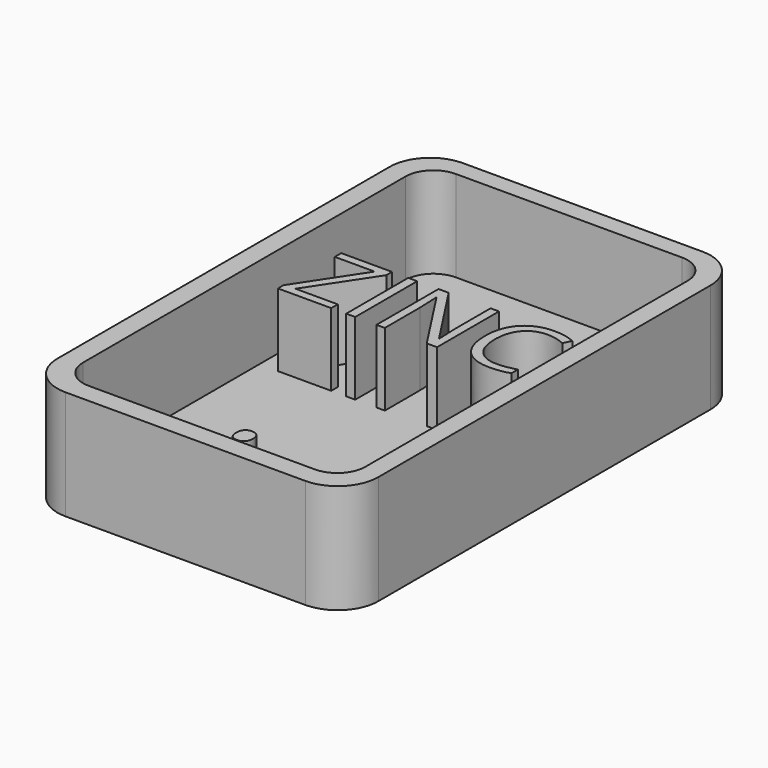
from build123d import *

# Parameters (mm, degrees)
F0_W         = 58.2063253969
F0_H         = 90.0586508214
F1_DEPTH     = 19.812
F2_W         = 51.1912312359
F2_H         = 83.2331553102
F3_DEPTH     = 16.51
F4_R         = 7.3585229381
F5_R         = 5.08
F6_TEXT_SIZE = 19.6911226441
F7_DEPTH     = 13.208
F8_TEXT_SIZE = 25.8062836818
F9_DEPTH     = 9.398


# Not quite as in the source:
# - Text() gives the source's letters only with a copy of the font that has no kerning and outlines rounded to 1/6400 em; it was checked with that copy


with BuildPart() as f1:
    # F0 (on Top) → F1 (new body)
    with BuildSketch(Plane.XY):
        with Locations((7.3942886665, -3.6023464054)):
            Rectangle(F0_W, F0_H)
    extrude(amount=F1_DEPTH)

    # F2 (on face) → F3 (cut)
    with BuildSketch(Plane.XY.offset(19.812)):
        with Locations((7.4890861288, -3.4127496183)):
            Rectangle(F2_W, F2_H)
    extrude(amount=-F3_DEPTH, mode=Mode.SUBTRACT)

    # F4
    f4_edges = [f1.edges().sort_by_distance(p)[0] for p in [
        (36.497451, -48.631672, 9.906),
        (-21.708874, -48.631672, 9.906),
        (-21.708874, 41.426979, 9.906),
        (36.497451, 41.426979, 9.906),
    ]]
    fillet(f4_edges, radius=F4_R)

    # F5
    f5_edges = [f1.edges().sort_by_distance(p)[0] for p in [
        (33.084702, 38.203828, 11.557),
        (-18.106529, 38.203828, 11.557),
        (-18.106529, -45.029327, 11.557),
        (33.084702, -45.029327, 11.557),
    ]]
    fillet(f5_edges, radius=F5_R)

    # F6 (on face) → F7 (join)
    with BuildSketch(Plane.XY.offset(3.302)):
        with Locations((-15.510027653, 0)):
            Text('ZINC', F6_TEXT_SIZE, font='Open Sans', text_align=(TextAlign.LEFT, TextAlign.BOTTOM))
    extrude(amount=F7_DEPTH)

    # F8 (on face) → F9 (join)
    with BuildSketch(Plane.XY.offset(3.302)):
        with Locations((1.8011715729, -33.8430907577)):
            Text('.', F8_TEXT_SIZE, font='Open Sans', text_align=(TextAlign.LEFT, TextAlign.BOTTOM))
    extrude(amount=F9_DEPTH)


solid = f1.part
